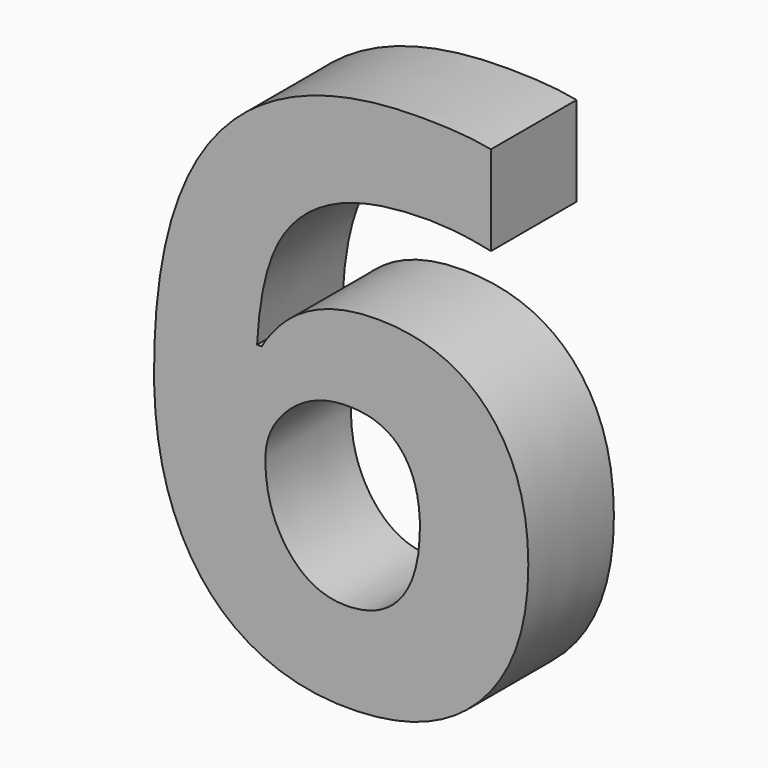
from build123d import *

# Parameters (mm, degrees)
F0_TEXT_SIZE = 35.2777777778
F1_DEPTH     = 5.08


# Not quite as in the source:
# - Text() gives the source's letters only with a copy of the font that has no kerning and outlines rounded to 1/6400 em; it was checked with that copy


with BuildPart() as f1:
    # F0 (on Front) → F1 (new body)
    with BuildSketch(Plane.XZ):
        with Locations((-65.6222173577, 26.9704465183)):
            Text('6', F0_TEXT_SIZE, font='Open Sans', font_style=FontStyle.BOLD, text_align=(TextAlign.LEFT, TextAlign.BOTTOM))
    extrude(amount=F1_DEPTH)


solid = f1.part
